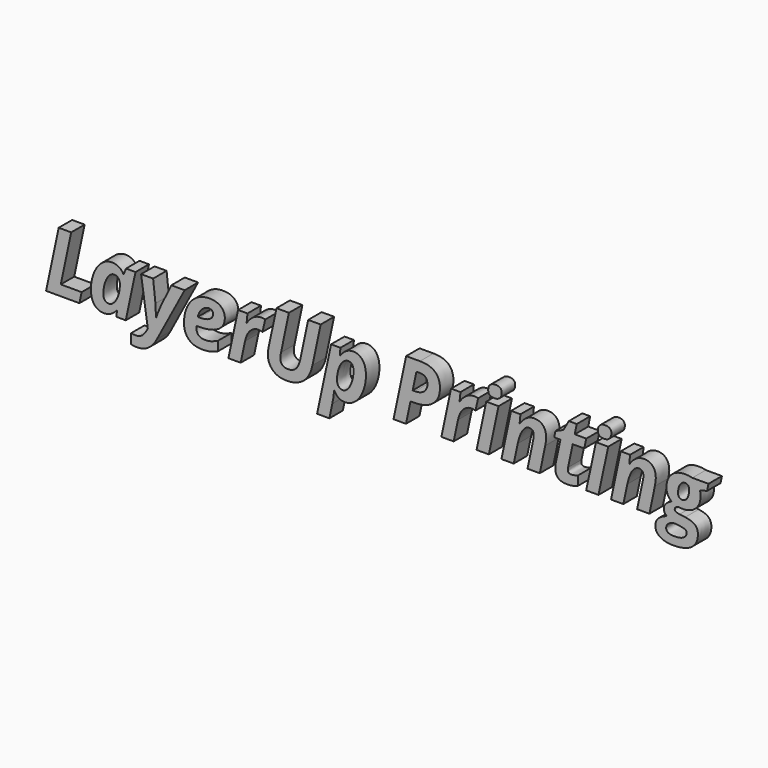
from build123d import *

# Parameters (mm, degrees)
F0_TEXT_SIZE = 12.6123480085
F1_DEPTH     = 2.54


# Not quite as in the source:
# - Text() gives the source's letters only with a copy of the font that has no kerning and outlines rounded to 1/6400 em; it was checked with that copy


with BuildPart() as f1:
    # F0 (on Front) → F1 (new body)
    with BuildSketch(Plane.XZ):
        with Locations((-62.9526525736, 17.9163496941)):
            Text('LayerUp Printing', F0_TEXT_SIZE, font='Open Sans', font_style=FontStyle.BOLDITALIC, text_align=(TextAlign.LEFT, TextAlign.BOTTOM))
    extrude(amount=F1_DEPTH)


solid = f1.part
